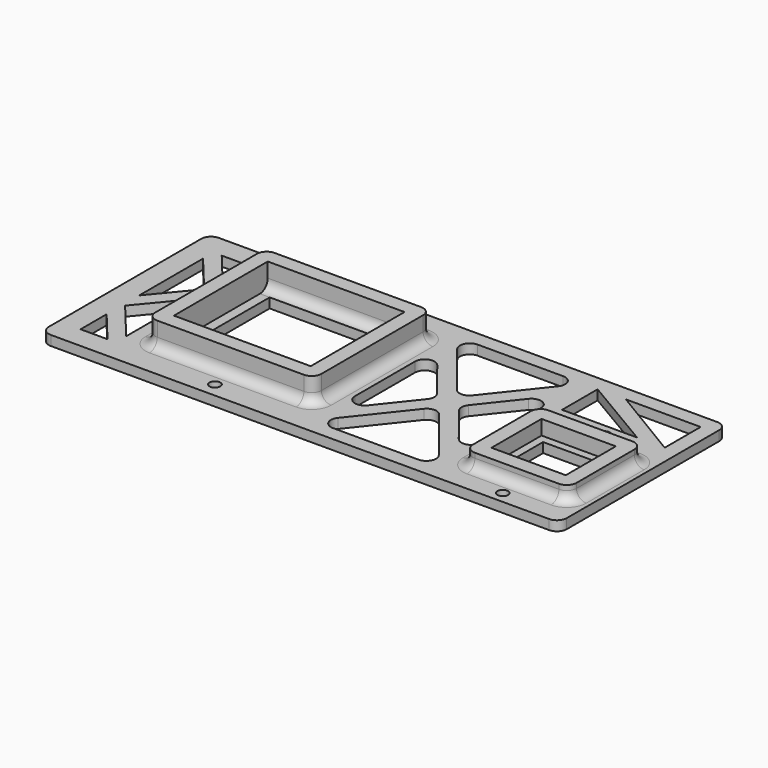
from build123d import *

# Parameters (mm, degrees)
F0_W     = 134.62
F0_H     = 54.61
F1_DEPTH = 2.54
F2_R     = 1.397
F3_DEPTH = 2.541
F2_W     = 43.18
F2_H     = 38.1
F2_W_2   = 35.56
F2_H_2   = 30.48
F4_DEPTH = 6.35
F2_W_3   = 26.924
F2_H_3   = 23.876
F2_W_4   = 19.304
F2_H_4   = 16.256
F5_DEPTH = 3.81
F6_W     = 30.48
F6_H     = 25.4
F6_W_2   = 15.24
F6_H_2   = 12.192
F7_DEPTH = 2.541
F8_R     = 2.53999
F9_R     = 2.54


# Not quite as in the source:
# - a fillet or chamfer is up to 0.001 mm smaller than in the source, because OpenCascade refuses the exact size
# - a feature names something its author has since deleted; it is built from what else it names


with BuildPart() as f1:
    # F0 (on Top) → F1 (new body)
    with BuildSketch(Plane.XY):
        Rectangle(F0_W, F0_H)
    extrude(amount=-F1_DEPTH)

    # F2 (on face) → F3 (cut, through all)
    with BuildSketch(Plane.XY):
        with Locations((-25.146, 24.765)):
            Circle(F2_R)
        with Locations((-25.146, -23.495)):
            Circle(F2_R)
        with Locations((50.292, 8.763)):
            Circle(F2_R)
        with Locations((50.292, -24.257)):
            Circle(F2_R)
    extrude(amount=-F3_DEPTH, mode=Mode.SUBTRACT)

    # F2 (on face) → F4 (join)
    with BuildSketch(Plane.XY):
        with Locations((-25.146, 0.635)):
            Rectangle(F2_W, F2_H)
        with Locations((-25.146, 0.635)):
            Rectangle(F2_W_2, F2_H_2, mode=Mode.SUBTRACT)
    extrude(amount=F4_DEPTH)

    # F2 (on face) → F5 (join)
    with BuildSketch(Plane.XY):
        with Locations((50.292, -7.747)):
            Rectangle(F2_W_3, F2_H_3)
        with Locations((50.292, -7.747)):
            Rectangle(F2_W_4, F2_H_4, mode=Mode.SUBTRACT)
    extrude(amount=F5_DEPTH)

    # F6 (on face) → F7 (cut, through all)
    with BuildSketch(Plane.XY):
        Polygon((13.7795, 0), (0.254, 17.0379360465), (0.254, -17.0379360465), align=None)
        Polygon((33.02, 23.495), (0.254, 23.495), (16.637, 2.8575), align=None)
        Polygon((33.02, -17.0379360465), (33.02, 17.0379360465), (19.4945, 0), align=None)
        Polygon((16.637, -2.8575), (0.254, -23.495), (33.02, -23.495), align=None)
        Polygon((56.3291969075, 11.811), (36.83, 23.3617037719), (36.83, 11.811), align=None)
        Polygon((63.5, 23.495), (44.0803815263, 23.495), (63.5, 11.811), align=None)
        with Locations((-25.146, 0.635)):
            Rectangle(F6_W, F6_H)
        with Locations((50.292, -7.747)):
            Rectangle(F6_W_2, F6_H_2)
        Polygon((-53.0180806356, 7.8316666667), (-61.595, 18.202451519), (-61.595, -2.5391181857), align=None)
        Polygon((-52.451, 21.59), (-59.4524328779, 21.59), (-52.451, 13.1242151477), align=None)
        Polygon((-52.451, -18.202451519), (-52.451, 2.5391181857), (-61.0279193644, -7.8316666667), align=None)
        Polygon((-54.5935671221, -21.59), (-61.595, -13.1242151477), (-61.595, -21.59), align=None)
    extrude(amount=-F7_DEPTH, mode=Mode.SUBTRACT)

    # F8 (radius 2.54 in the source; OpenCascade refuses exactly that, so slightly less here)
    f8_edges = [f1.edges().sort_by_distance(p)[0] for p in [
        (-25.146, -18.415, 0),
        (-46.736, 0.635, 0),
        (50.292, -19.685, 0),
        (36.83, -7.747, 0),
        (-25.146, 19.685, 0),
        (-3.556, 0.635, 0),
        (63.754, -7.747, 0),
        (50.292, 4.191, 0),
        (63.754, 4.191, 1.905),
        (63.754, -19.685, 1.905),
        (-3.556, 19.685, 3.175),
        (-3.556, -18.415, 3.175),
        (36.83, -19.685, 1.905),
        (-46.736, -18.415, 3.175),
        (-46.736, 19.685, 3.175),
        (36.83, 4.191, 1.905),
        (-25.146, 15.875, 0),
        (-25.146, -14.605, 0),
        (-67.31, -27.305, -1.27),
        (-67.31, 27.305, -1.27),
        (67.31, 27.305, -1.27),
        (67.31, -27.305, -1.27),
    ]]
    fillet(f8_edges, radius=F8_R)

    # F9
    f9_edges = [f1.edges().sort_by_distance(p)[0] for p in [
        (33.02, 23.495, -1.27),
        (13.7795, 0, -1.27),
        (16.637, -2.8575, -1.27),
        (0.254, 17.037936, -1.27),
        (33.02, 17.037936, -1.27),
        (33.02, -17.037936, -1.27),
        (33.02, -23.495, -1.27),
        (0.254, 23.495, -1.27),
        (0.254, -23.495, -1.27),
        (0.254, -17.037936, -1.27),
        (19.4945, 0, -1.27),
        (16.637, 2.8575, -1.27),
    ]]
    fillet(f9_edges, radius=F9_R)


solid = f1.part
